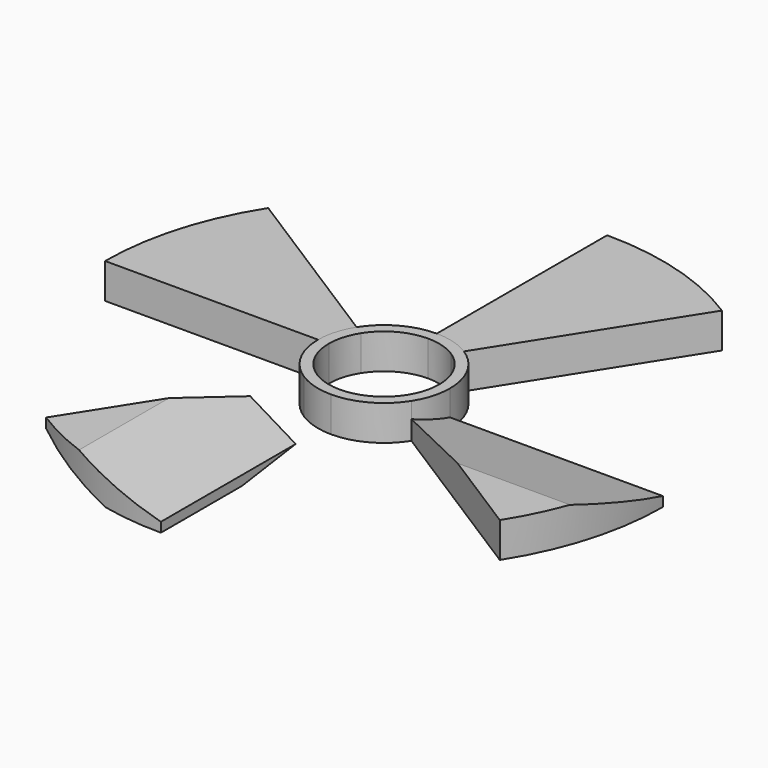
from build123d import *

# Parameters (mm, degrees)
F1_DEPTH    = 7
F2_DEPTH    = 7
F3_SIZE2    = 18.9588181024
F3_SIZE     = 5.08
F3_2_SIZE2  = 18.9588181024
F3_2_SIZE   = 5.08
F4_T1_DEPTH = 140.8854077886


# Not quite as in the source:
# - a fillet or chamfer that OpenCascade refuses, or shapes differently, is made with other operations: its cross-section is extruded or revolved along the edge and cut away or added


with BuildPart() as f1:
    # F0 (on Top) → F1 (new body)
    with BuildSketch(Plane.XY):
        with BuildLine():
            Line((-13.1396949858, 0), (-11, 0))
            ThreePointArc((-11, 0), (-10.5625846979, 3.0711243054), (-9.2851264546, 5.8980019262))
            Line((-9.2851264546, 5.8980019262), (-11.0912481381, 7.0452678487))
            ThreePointArc((-11.0912481381, 7.0452678487), (-12.6171946539, 3.6685124216), (-13.1396949858, 0))
        make_face()
        with BuildLine():
            ThreePointArc((-9.2851264546, 5.8980019262), (-5.2972624445, 9.640488089), (0, 11))
            Line((0, 11), (0, 13.1396949858))
            ThreePointArc((0, 13.1396949858), (-6.3276738891, 11.5157339094), (-11.0912481381, 7.0452678487))
            Line((-11.0912481381, 7.0452678487), (-9.2851264546, 5.8980019262))
        make_face()
        with BuildLine():
            ThreePointArc((0, 11), (3.0711243054, 10.5625846979), (5.8980019262, 9.2851264546))
            Line((5.8980019262, 9.2851264546), (7.0452678487, 11.0912481381))
            ThreePointArc((7.0452678487, 11.0912481381), (3.6685124216, 12.6171946539), (0, 13.1396949858))
            Line((0, 13.1396949858), (0, 11))
        make_face()
        with BuildLine():
            ThreePointArc((5.8980019262, 9.2851264546), (9.640488089, 5.2972624445), (11, 0))
            Line((11, 0), (13.1396949858, 0))
            ThreePointArc((13.1396949858, 0), (11.5157339094, 6.3276738891), (7.0452678487, 11.0912481381))
            Line((7.0452678487, 11.0912481381), (5.8980019262, 9.2851264546))
        make_face()
        with BuildLine():
            Line((13.1396949858, 0), (11, 0))
            ThreePointArc((11, 0), (10.5625846979, -3.0711243054), (9.2851264546, -5.8980019262))
            Line((9.2851264546, -5.8980019262), (11.0912481381, -7.0452678487))
            ThreePointArc((11.0912481381, -7.0452678487), (12.6171946539, -3.6685124216), (13.1396949858, 0))
        make_face()
        with BuildLine():
            Line((11.0912481381, -7.0452678487), (9.2851264546, -5.8980019262))
            ThreePointArc((9.2851264546, -5.8980019262), (5.2972624445, -9.640488089), (0, -11))
            Line((0, -11), (0, -13.1396949858))
            ThreePointArc((0, -13.1396949858), (6.3276738891, -11.5157339094), (11.0912481381, -7.0452678487))
        make_face()
        with BuildLine():
            Line((0, -13.1396949858), (0, -11))
            ThreePointArc((0, -11), (-3.0711243054, -10.5625846979), (-5.8980019262, -9.2851264546))
            Line((-5.8980019262, -9.2851264546), (-7.0452678487, -11.0912481381))
            ThreePointArc((-7.0452678487, -11.0912481381), (-3.6685124216, -12.6171946539), (0, -13.1396949858))
        make_face()
        with BuildLine():
            ThreePointArc((-5.8980019262, -9.2851264546), (-9.640488089, -5.2972624445), (-11, 0))
            Line((-11, 0), (-13.1396949858, 0))
            ThreePointArc((-13.1396949858, 0), (-11.5157339094, -6.3276738891), (-7.0452678487, -11.0912481381))
            Line((-7.0452678487, -11.0912481381), (-5.8980019262, -9.2851264546))
        make_face()
    extrude(amount=F1_DEPTH)


with BuildPart() as f2:
    # F0 (on Top) → F2 (new body)
    with BuildSketch(Plane.XY):
        with BuildLine():
            ThreePointArc((0, 13.1396949858), (3.6685124216, 12.6171946539), (7.0452678487, 11.0912481381))
            Line((7.0452678487, 11.0912481381), (29.7921797922, 46.9013337383))
            Line((29.7921797922, 46.9013337383), (0, 53.34))
            Line((0, 53.34), (0, 13.1396949858))
        make_face()
        with BuildLine():
            Line((0, 53.34), (29.7921797922, 46.9013337383))
            ThreePointArc((29.7921797922, 46.9013337383), (15.5129633081, 53.3540725025), (0, 55.5635589501))
            Line((0, 55.5635589501), (0, 53.34))
        make_face()
    extrude(amount=F2_DEPTH)


with BuildPart() as f2b:
    # F0 (on Top) → F2, piece 2 (new body)
    with BuildSketch(Plane.XY):
        with BuildLine():
            Line((-53.34, 0), (-13.1396949858, 0))
            ThreePointArc((-13.1396949858, 0), (-12.6171946539, 3.6685124216), (-11.0912481381, 7.0452678487))
            Line((-11.0912481381, 7.0452678487), (-46.9013337383, 29.7921797922))
            Line((-46.9013337383, 29.7921797922), (-53.34, 0))
        make_face()
        with BuildLine():
            Line((-55.5635589501, 0), (-53.34, 0))
            Line((-53.34, 0), (-46.9013337383, 29.7921797922))
            ThreePointArc((-46.9013337383, 29.7921797922), (-53.3540725025, 15.5129633081), (-55.5635589501, 0))
        make_face()
    extrude(amount=F2_DEPTH)


with BuildPart() as f2c:
    # F0 (on Top) → F2, piece 3 (new body)
    with BuildSketch(Plane.XY):
        with BuildLine():
            Line((0, -53.34), (0, -13.1396949858))
            ThreePointArc((0, -13.1396949858), (-3.6685124216, -12.6171946539), (-7.0452678487, -11.0912481381))
            Line((-7.0452678487, -11.0912481381), (-29.7921797922, -46.9013337383))
            Line((-29.7921797922, -46.9013337383), (0, -53.34))
        make_face()
        with BuildLine():
            Line((0, -55.5635589501), (0, -53.34))
            Line((0, -53.34), (-29.7921797922, -46.9013337383))
            ThreePointArc((-29.7921797922, -46.9013337383), (-15.5129633081, -53.3540725025), (0, -55.5635589501))
        make_face()
    extrude(amount=F2_DEPTH)

    # F3
    f3_edges = [f2c.edges().sort_by_distance(p)[0] for p in [
        (0, -34.351627, 7),
    ]]
    f3_side = f2c.faces().sort_by_distance((0, -34.351627, 3.5))[0]
    chamfer(f3_edges, length=F3_SIZE, length2=F3_SIZE2, reference=f3_side)

    # F4: chamfer of 5.08 x 18.9588181024 on 1 edges, made by hand

    # F4_s2 → F4_t1 (cut)
    with BuildSketch(Plane(origin=(19.3513855664, 30.4645648313, 0), x_dir=(0, 0, 1), z_dir=(-0.5361819933, -0.844102405, 0))):
        Polygon((5.08, 0), (0, -18.9588181024), (0, 0), align=None)
    extrude(amount=F4_T1_DEPTH, mode=Mode.SUBTRACT)


with BuildPart() as f2d:
    # F0 (on Top) → F2, piece 4 (new body)
    with BuildSketch(Plane.XY):
        with BuildLine():
            Line((53.34, 0), (13.1396949858, 0))
            ThreePointArc((13.1396949858, 0), (12.6171946539, -3.6685124216), (11.0912481381, -7.0452678487))
            Line((11.0912481381, -7.0452678487), (46.9013337383, -29.7921797922))
            Line((46.9013337383, -29.7921797922), (53.34, 0))
        make_face()
        with BuildLine():
            Line((55.5635589501, 0), (53.34, 0))
            Line((53.34, 0), (46.9013337383, -29.7921797922))
            ThreePointArc((46.9013337383, -29.7921797922), (53.3540725025, -15.5129633081), (55.5635589501, 0))
        make_face()
    extrude(amount=F2_DEPTH)

    # F3#2
    f3_2_edges = [f2d.edges().sort_by_distance(p)[0] for p in [
        (34.351627, 0, 7),
    ]]
    f3_2_side = f2d.faces().sort_by_distance((34.351627, 0, 3.5))[0]
    chamfer(f3_2_edges, length=F3_2_SIZE, length2=F3_2_SIZE2, reference=f3_2_side)


solid = Compound([f1.part, f2.part, f2b.part, f2c.part, f2d.part])
